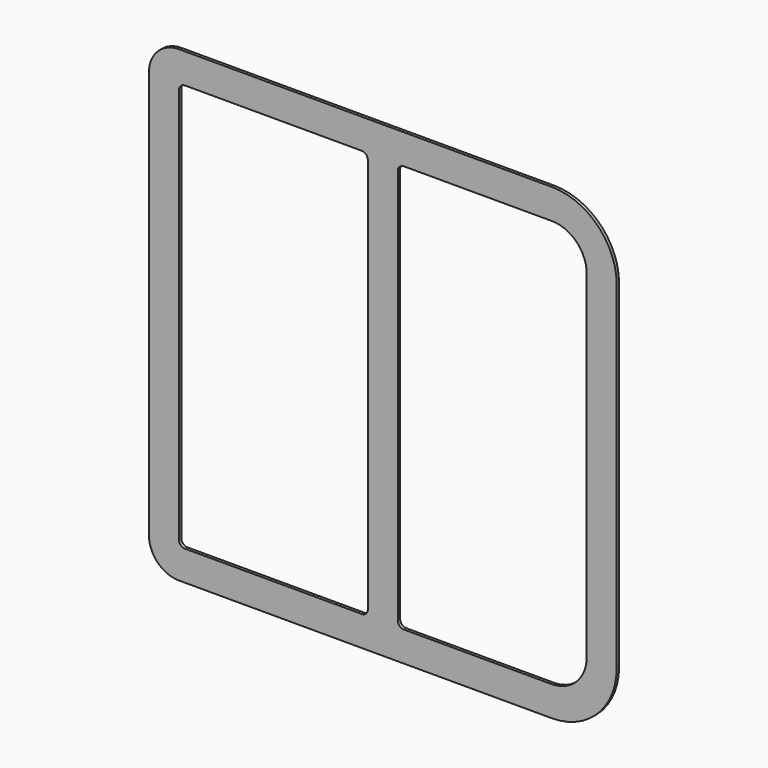
from build123d import *

# Parameters (mm, degrees)
F1_DEPTH = 3
F2_DEPTH = 2


# Not quite as in the source:
# - a feature names something its author has since deleted; it is built from what else it names


with BuildPart() as f1:
    # F0 (on Front) → F1 (new body)
    with BuildSketch(Plane.XZ):
        with BuildLine():
            Line((-185.9730800638, 26.8439535797), (-185.9730800638, 364.8439535797))
            ThreePointArc((-185.9730800638, 364.8439535797), (-205.0111392867, 410.8058943568), (-250.9730800638, 429.8439535797))
            Line((-250.9730800638, 429.8439535797), (-623.9730800638, 429.8439535797))
            ThreePointArc((-623.9730800638, 429.8439535797), (-645.1862834994, 421.0571570153), (-653.9730800638, 399.8439535797))
            Line((-653.9730800638, 399.8439535797), (-653.9730800638, -8.1560464203))
            ThreePointArc((-653.9730800638, -8.1560464203), (-645.1862834994, -29.3692498559), (-623.9730800638, -38.1560464203))
            Line((-623.9730800638, -38.1560464203), (-250.9730800638, -38.1560464203))
            ThreePointArc((-250.9730800638, -38.1560464203), (-205.0111392867, -19.1179871975), (-185.9730800638, 26.8439535797))
        make_face()
        with BuildLine():
            ThreePointArc((-637.9730800638, 414.1268104367), (-631.5342592992, 418.3595839651), (-623.9730800638, 419.8439535797))
            Line((-623.9730800638, 419.8439535797), (-250.9730800638, 419.8439535797))
            ThreePointArc((-250.9730800638, 419.8439535797), (-229.9254912838, 415.6573278678), (-212.0822070986, 403.7348265449))
            ThreePointArc((-212.0822070986, 403.7348265449), (-200.1597057757, 385.8915423597), (-195.9730800638, 364.8439535797))
            Line((-195.9730800638, 364.8439535797), (-195.9730800638, 195.8439535797))
            Line((-195.9730800638, 195.8439535797), (-195.9730800638, 26.8439535797))
            ThreePointArc((-195.9730800638, 26.8439535797), (-200.1597057757, 5.7963647996), (-212.0822070986, -12.0469193856))
            ThreePointArc((-212.0822070986, -12.0469193856), (-229.9254912838, -23.9694207085), (-250.9730800638, -28.1560464203))
            Line((-250.9730800638, -28.1560464203), (-623.9730800638, -28.1560464203))
            ThreePointArc((-623.9730800638, -28.1560464203), (-631.6267487111, -26.6336370706), (-638.1152156876, -22.2981820441))
            ThreePointArc((-638.1152156876, -22.2981820441), (-642.4506707141, -15.8097150676), (-643.9730800638, -8.1560464203))
            Line((-643.9730800638, -8.1560464203), (-643.9730800638, 195.8439535797))
            Line((-643.9730800638, 195.8439535797), (-643.9730800638, 399.8439535797))
            ThreePointArc((-643.9730800638, 399.8439535797), (-642.4121689784, 407.5899202721), (-637.9730800638, 414.1268104367))
        make_face(mode=Mode.SUBTRACT)
        with BuildLine():
            ThreePointArc((-623.9730800638, 413.8439535797), (-629.330648117, 412.7782670348), (-633.8725750005, 409.7434485163))
            ThreePointArc((-633.8725750005, 409.7434485163), (-636.907393519, 405.2015216328), (-637.9730800638, 399.8439535797))
            Line((-637.9730800638, 399.8439535797), (-637.9730800638, 195.8439535797))
            Line((-637.9730800638, 195.8439535797), (-637.9730800638, -8.1560464203))
            ThreePointArc((-637.9730800638, -8.1560464203), (-636.907393519, -13.5136144734), (-633.8725750005, -18.0555413569))
            ThreePointArc((-633.8725750005, -18.0555413569), (-629.330648117, -21.0903598755), (-623.9730800638, -22.1560464203))
            Line((-623.9730800638, -22.1560464203), (-428.9730800638, -22.1560464203))
            ThreePointArc((-428.9730800638, -22.1560464203), (-424.7304393767, -20.3986871075), (-422.9730800638, -16.1560464203))
            Line((-422.9730800638, -16.1560464203), (-422.9730800638, 407.8439535797))
            ThreePointArc((-422.9730800638, 407.8439535797), (-424.7304393767, 412.0865942668), (-428.9730800638, 413.8439535797))
            Line((-428.9730800638, 413.8439535797), (-623.9730800638, 413.8439535797))
        make_face()
        with BuildLine():
            Line((-623.9730800638, -2.1560464203), (-623.9730800638, 393.8439535797))
            ThreePointArc((-623.9730800638, 393.8439535797), (-622.215720751, 398.0865942668), (-617.9730800638, 399.8439535797))
            Line((-617.9730800638, 399.8439535797), (-440.9730800638, 399.8439535797))
            ThreePointArc((-440.9730800638, 399.8439535797), (-436.7304393767, 398.0865942668), (-434.9730800638, 393.8439535797))
            Line((-434.9730800638, 393.8439535797), (-434.9730800638, -2.1560464203))
            ThreePointArc((-434.9730800638, -2.1560464203), (-436.7304393767, -6.3986871075), (-440.9730800638, -8.1560464203))
            Line((-440.9730800638, -8.1560464203), (-617.9730800638, -8.1560464203))
            ThreePointArc((-617.9730800638, -8.1560464203), (-622.215720751, -6.3986871075), (-623.9730800638, -2.1560464203))
        make_face(mode=Mode.SUBTRACT)
        with BuildLine():
            ThreePointArc((-201.9730800638, 364.8439535797), (-205.7029829708, 383.5954417656), (-216.3248477857, 399.4921858578))
            ThreePointArc((-216.3248477857, 399.4921858578), (-232.221591878, 410.1140506727), (-250.9730800638, 413.8439535797))
            Line((-250.9730800638, 413.8439535797), (-410.9730800638, 413.8439535797))
            ThreePointArc((-410.9730800638, 413.8439535797), (-415.215720751, 412.0865942668), (-416.9730800638, 407.8439535797))
            Line((-416.9730800638, 407.8439535797), (-416.9730800638, -16.1560464203))
            ThreePointArc((-416.9730800638, -16.1560464203), (-415.215720751, -20.3986871075), (-410.9730800638, -22.1560464203))
            Line((-410.9730800638, -22.1560464203), (-250.9730800638, -22.1560464203))
            ThreePointArc((-250.9730800638, -22.1560464203), (-232.221591878, -18.4261435134), (-216.3248477857, -7.8042786985))
            ThreePointArc((-216.3248477857, -7.8042786985), (-205.7029829708, 8.0924653938), (-201.9730800638, 26.8439535797))
            Line((-201.9730800638, 26.8439535797), (-201.9730800638, 195.8439535797))
            Line((-201.9730800638, 195.8439535797), (-201.9730800638, 364.8439535797))
        make_face()
        with BuildLine():
            ThreePointArc((-404.9730800638, 393.8439535797), (-403.215720751, 398.0865942668), (-398.9730800638, 399.8439535797))
            Line((-398.9730800638, 399.8439535797), (-250.9730800638, 399.8439535797))
            ThreePointArc((-250.9730800638, 399.8439535797), (-226.2243427223, 389.5926909212), (-215.9730800638, 364.8439535797))
            Line((-215.9730800638, 364.8439535797), (-215.9730800638, 26.8439535797))
            ThreePointArc((-215.9730800638, 26.8439535797), (-226.2243427223, 2.0952162381), (-250.9730800638, -8.1560464203))
            Line((-250.9730800638, -8.1560464203), (-398.9730800638, -8.1560464203))
            ThreePointArc((-398.9730800638, -8.1560464203), (-403.215720751, -6.3986871075), (-404.9730800638, -2.1560464203))
            Line((-404.9730800638, -2.1560464203), (-404.9730800638, 393.8439535797))
        make_face(mode=Mode.SUBTRACT)
        with BuildLine():
            Line((-250.9730800638, 419.8439535797), (-623.9730800638, 419.8439535797))
            ThreePointArc((-623.9730800638, 419.8439535797), (-631.5342592992, 418.3595839651), (-637.9730800638, 414.1268104367))
            Line((-637.9730800638, 414.1268104367), (-633.8725750005, 409.7434485163))
            ThreePointArc((-633.8725750005, 409.7434485163), (-629.330648117, 412.7782670348), (-623.9730800638, 413.8439535797))
            Line((-623.9730800638, 413.8439535797), (-428.9730800638, 413.8439535797))
            ThreePointArc((-428.9730800638, 413.8439535797), (-424.7304393767, 412.0865942668), (-422.9730800638, 407.8439535797))
            Line((-422.9730800638, 407.8439535797), (-422.9730800638, -16.1560464203))
            ThreePointArc((-422.9730800638, -16.1560464203), (-424.7304393767, -20.3986871075), (-428.9730800638, -22.1560464203))
            Line((-428.9730800638, -22.1560464203), (-623.9730800638, -22.1560464203))
            ThreePointArc((-623.9730800638, -22.1560464203), (-629.330648117, -21.0903598755), (-633.8725750005, -18.0555413569))
            Line((-633.8725750005, -18.0555413569), (-638.1152156876, -22.2981820441))
            ThreePointArc((-638.1152156876, -22.2981820441), (-631.6267487111, -26.6336370706), (-623.9730800638, -28.1560464203))
            Line((-623.9730800638, -28.1560464203), (-250.9730800638, -28.1560464203))
            ThreePointArc((-250.9730800638, -28.1560464203), (-229.9254912838, -23.9694207085), (-212.0822070986, -12.0469193856))
            Line((-212.0822070986, -12.0469193856), (-216.3248477857, -7.8042786985))
            ThreePointArc((-216.3248477857, -7.8042786985), (-232.221591878, -18.4261435134), (-250.9730800638, -22.1560464203))
            Line((-250.9730800638, -22.1560464203), (-410.9730800638, -22.1560464203))
            ThreePointArc((-410.9730800638, -22.1560464203), (-415.215720751, -20.3986871075), (-416.9730800638, -16.1560464203))
            Line((-416.9730800638, -16.1560464203), (-416.9730800638, 407.8439535797))
            ThreePointArc((-416.9730800638, 407.8439535797), (-415.215720751, 412.0865942668), (-410.9730800638, 413.8439535797))
            Line((-410.9730800638, 413.8439535797), (-250.9730800638, 413.8439535797))
            ThreePointArc((-250.9730800638, 413.8439535797), (-232.221591878, 410.1140506727), (-216.3248477857, 399.4921858578))
            Line((-216.3248477857, 399.4921858578), (-212.0822070986, 403.7348265449))
            ThreePointArc((-212.0822070986, 403.7348265449), (-229.9254912838, 415.6573278678), (-250.9730800638, 419.8439535797))
        make_face()
        with BuildLine():
            Line((-633.8725750005, 409.7434485163), (-637.9730800638, 414.1268104367))
            ThreePointArc((-637.9730800638, 414.1268104367), (-642.4121689784, 407.5899202721), (-643.9730800638, 399.8439535797))
            Line((-643.9730800638, 399.8439535797), (-643.9730800638, 195.8439535797))
            Line((-643.9730800638, 195.8439535797), (-637.9730800638, 195.8439535797))
            Line((-637.9730800638, 195.8439535797), (-637.9730800638, 399.8439535797))
            ThreePointArc((-637.9730800638, 399.8439535797), (-636.907393519, 405.2015216328), (-633.8725750005, 409.7434485163))
        make_face()
        with BuildLine():
            Line((-637.9730800638, 195.8439535797), (-643.9730800638, 195.8439535797))
            Line((-643.9730800638, 195.8439535797), (-643.9730800638, -8.1560464203))
            ThreePointArc((-643.9730800638, -8.1560464203), (-642.4506707141, -15.8097150676), (-638.1152156876, -22.2981820441))
            Line((-638.1152156876, -22.2981820441), (-633.8725750005, -18.0555413569))
            ThreePointArc((-633.8725750005, -18.0555413569), (-636.907393519, -13.5136144734), (-637.9730800638, -8.1560464203))
            Line((-637.9730800638, -8.1560464203), (-637.9730800638, 195.8439535797))
        make_face()
        with BuildLine():
            ThreePointArc((-195.9730800638, 364.8439535797), (-200.1597057757, 385.8915423597), (-212.0822070986, 403.7348265449))
            Line((-212.0822070986, 403.7348265449), (-216.3248477857, 399.4921858578))
            ThreePointArc((-216.3248477857, 399.4921858578), (-205.7029829708, 383.5954417656), (-201.9730800638, 364.8439535797))
            Line((-201.9730800638, 364.8439535797), (-201.9730800638, 195.8439535797))
            Line((-201.9730800638, 195.8439535797), (-195.9730800638, 195.8439535797))
            Line((-195.9730800638, 195.8439535797), (-195.9730800638, 364.8439535797))
        make_face()
        with BuildLine():
            Line((-195.9730800638, 26.8439535797), (-195.9730800638, 195.8439535797))
            Line((-195.9730800638, 195.8439535797), (-201.9730800638, 195.8439535797))
            Line((-201.9730800638, 195.8439535797), (-201.9730800638, 26.8439535797))
            ThreePointArc((-201.9730800638, 26.8439535797), (-205.7029829708, 8.0924653938), (-216.3248477857, -7.8042786985))
            Line((-216.3248477857, -7.8042786985), (-212.0822070986, -12.0469193856))
            ThreePointArc((-212.0822070986, -12.0469193856), (-200.1597057757, 5.7963647996), (-195.9730800638, 26.8439535797))
        make_face()
    extrude(amount=F1_DEPTH)

    # F0 (on Front) → F2 (join)
    with BuildSketch(Plane.XZ):
        with BuildLine():
            ThreePointArc((-195.9730800638, 364.8439535797), (-200.1597057757, 385.8915423597), (-212.0822070986, 403.7348265449))
            Line((-212.0822070986, 403.7348265449), (-216.3248477857, 399.4921858578))
            ThreePointArc((-216.3248477857, 399.4921858578), (-205.7029829708, 383.5954417656), (-201.9730800638, 364.8439535797))
            Line((-201.9730800638, 364.8439535797), (-201.9730800638, 195.8439535797))
            Line((-201.9730800638, 195.8439535797), (-195.9730800638, 195.8439535797))
            Line((-195.9730800638, 195.8439535797), (-195.9730800638, 364.8439535797))
        make_face()
        with BuildLine():
            Line((-195.9730800638, 26.8439535797), (-195.9730800638, 195.8439535797))
            Line((-195.9730800638, 195.8439535797), (-201.9730800638, 195.8439535797))
            Line((-201.9730800638, 195.8439535797), (-201.9730800638, 26.8439535797))
            ThreePointArc((-201.9730800638, 26.8439535797), (-205.7029829708, 8.0924653938), (-216.3248477857, -7.8042786985))
            Line((-216.3248477857, -7.8042786985), (-212.0822070986, -12.0469193856))
            ThreePointArc((-212.0822070986, -12.0469193856), (-200.1597057757, 5.7963647996), (-195.9730800638, 26.8439535797))
        make_face()
        with BuildLine():
            Line((-637.9730800638, 195.8439535797), (-643.9730800638, 195.8439535797))
            Line((-643.9730800638, 195.8439535797), (-643.9730800638, -8.1560464203))
            ThreePointArc((-643.9730800638, -8.1560464203), (-642.4506707141, -15.8097150676), (-638.1152156876, -22.2981820441))
            Line((-638.1152156876, -22.2981820441), (-633.8725750005, -18.0555413569))
            ThreePointArc((-633.8725750005, -18.0555413569), (-636.907393519, -13.5136144734), (-637.9730800638, -8.1560464203))
            Line((-637.9730800638, -8.1560464203), (-637.9730800638, 195.8439535797))
        make_face()
        with BuildLine():
            Line((-633.8725750005, 409.7434485163), (-637.9730800638, 414.1268104367))
            ThreePointArc((-637.9730800638, 414.1268104367), (-642.4121689784, 407.5899202721), (-643.9730800638, 399.8439535797))
            Line((-643.9730800638, 399.8439535797), (-643.9730800638, 195.8439535797))
            Line((-643.9730800638, 195.8439535797), (-637.9730800638, 195.8439535797))
            Line((-637.9730800638, 195.8439535797), (-637.9730800638, 399.8439535797))
            ThreePointArc((-637.9730800638, 399.8439535797), (-636.907393519, 405.2015216328), (-633.8725750005, 409.7434485163))
        make_face()
    extrude(amount=-F2_DEPTH)


solid = f1.part
